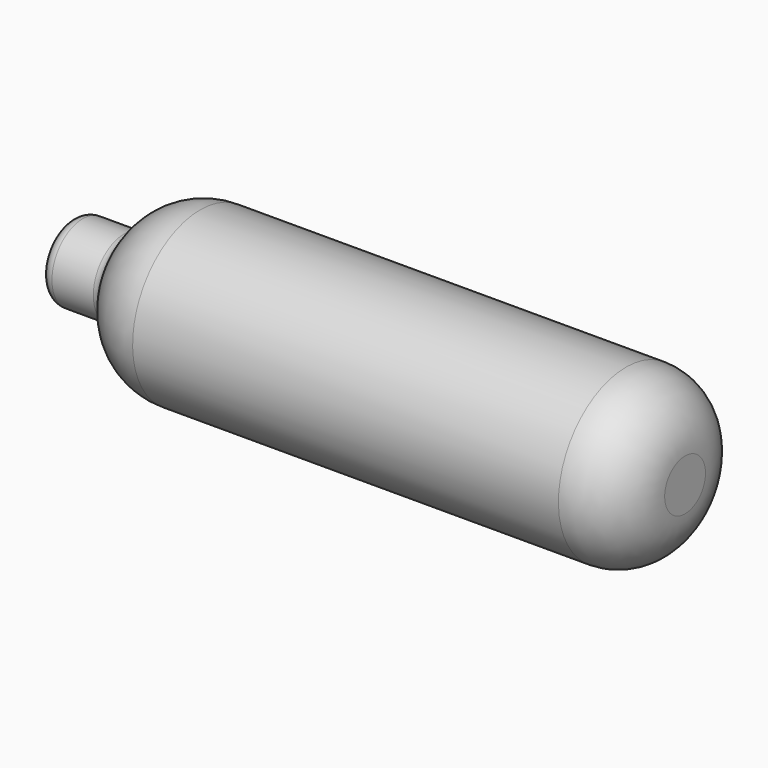
from build123d import *

# Parameters (mm, degrees)
F2_R = 6.096
F4_R = 1.27


# Not quite as in the source:
# - a fillet or chamfer that OpenCascade refuses, or shapes differently, is made with other operations: its cross-section is extruded or revolved along the edge and cut away or added


with BuildPart() as f1:
    # F0 (on Front) → F1 (revolve)
    with BuildSketch(Plane.XZ):
        Polygon((-25.6974867058, 3.96875), (-25.6974867058, 0), (37.8025132942, 0), (37.8025132942, 8.73125), (-19.3474867058, 8.73125), (-19.3474867058, 3.96875), align=None)
    revolve(axis=Axis((6.0525132942, 0, 0), (1, 0, 0)))

    # F2
    f2_edges = [f1.edges().sort_by_distance(p)[0] for p in [
        (37.802513, 0, -8.73125),
    ]]
    fillet(f2_edges, radius=F2_R)

    # F3: fillet of radius 7.62 on 1 edges, made by hand

    # F3_s1 → F3_t2 (revolve, cut)
    with BuildSketch(Plane.XZ):
        with BuildLine():
            ThreePointArc((-12.2835576468, 8.73125), (-16.543267144, 7.4294202256), (-19.3474867058, 3.96875))
            Line((-19.3474867058, 3.96875), (-19.3474867058, 8.73125))
            Line((-19.3474867058, 8.73125), (-12.2835576468, 8.73125))
        make_face()
    revolve(axis=Axis((-19.3474867058, 0, 0), (1, 0, 0)), mode=Mode.SUBTRACT)

    # F4
    f4_edges = [f1.edges().sort_by_distance(p)[0] for p in [
        (-22.522487, 0, 3.96875),
        (-25.697487, 0, -3.96875),
        (-19.347487, 0, -3.96875),
    ]]
    fillet(f4_edges, radius=F4_R)


solid = f1.part
